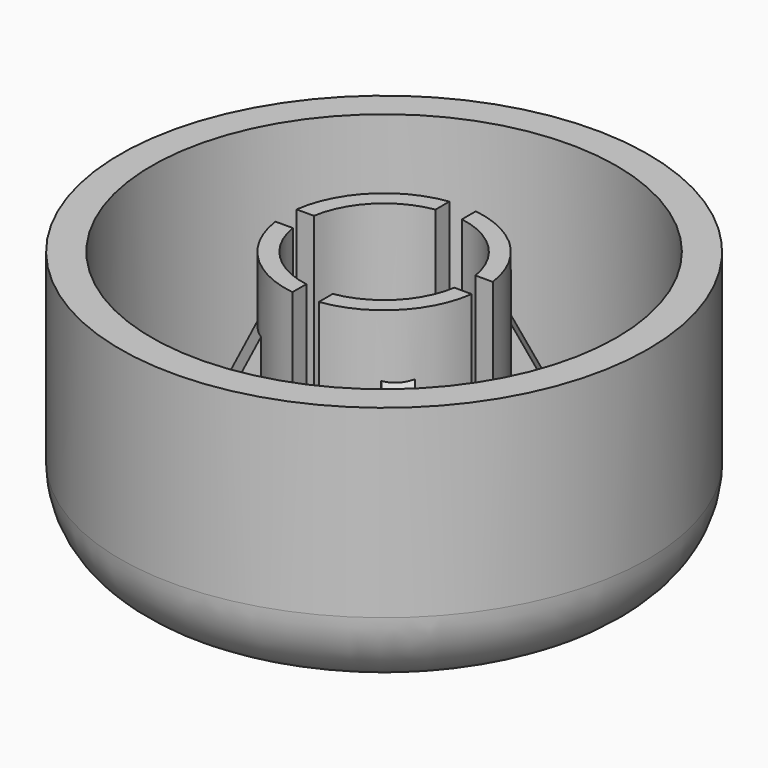
from build123d import *

# Parameters (mm, degrees)
F0_R         = 10
F0_R_2       = 3.1
F1_DEPTH     = 10
F2_R         = 8.8088832383
F2_R_2       = 3.75
F3_DEPTH     = 8
F4_W         = 1
F4_H         = 3.2863240922
F4_W_2       = 2.5055953301
F4_H_2       = 1
F5_DEPTH     = 7.5
F6_R         = 3
F8_DEPTH     = 6
F9_T4_DEPTH  = 1
F9_S5_R      = 3.75
F9_T6_DEPTH  = 5
F9_T10_DEPTH = 1
F9_S11_R     = 3.75
F9_T12_DEPTH = 5
F9_T16_DEPTH = 1
F9_S17_R     = 3.75
F9_T18_DEPTH = 5
F9_T22_DEPTH = 1
F9_S23_R     = 3.75
F9_T24_DEPTH = 5


# Not quite as in the source:
# - a fillet or chamfer that OpenCascade refuses, or shapes differently, is made with other operations: its cross-section is extruded or revolved along the edge and cut away or added
# - two fillets or chamfers of one size are made in one step


with BuildPart() as f1:
    # F0 (on Top) → F1 (new body)
    with BuildSketch(Plane.XY):
        Circle(F0_R)
        Circle(F0_R_2, mode=Mode.SUBTRACT)
    extrude(amount=F1_DEPTH)

    # F2 (on face) → F3 (cut)
    with BuildSketch(Plane.XY.offset(10)):
        Circle(F2_R)
        Circle(F2_R_2, mode=Mode.SUBTRACT)
    extrude(amount=-F3_DEPTH, mode=Mode.SUBTRACT)

    # F4 (on face) → F5 (cut)
    with BuildSketch(Plane.XY.offset(10)):
        Polygon((-2.7353764913, 0.5), (-4.8153767841, 0.5), (-4.8553765493, -0.5), (-2.7353764913, -0.5), align=None)
        Polygon((-0.5, 4.8884870484), (-0.5, 4.6887658536), (-0.5, 1.9834490959), (0.5, 1.9834490959), (0.5, 4.8884870484), align=None)
        with Locations((0, -3.2546973671)):
            Rectangle(F4_W, F4_H)
        with Locations((3.5874212626, 0)):
            Rectangle(F4_W_2, F4_H_2)
    extrude(amount=-F5_DEPTH, mode=Mode.SUBTRACT)

    # F6
    f6_edges = [f1.edges().sort_by_distance(p)[0] for p in [
        (-10, 0, 0),
    ]]
    fillet(f6_edges, radius=F6_R)

    # F7 (on face) → F8 (join)
    with BuildSketch(Plane.XY.offset(2)):
        Polygon((-4.9753358018, 4.2682290206), (-2.9815278958, 2.2744211146), (-2.2744211146, 2.9815278958), (-4.2682290206, 4.9753358018), align=None)
        Polygon((2.2744211146, 2.9815278958), (2.9815278958, 2.2744211146), (4.9753358018, 4.2682290206), (4.2682290206, 4.9753358018), align=None)
        Polygon((-2.2744211146, -2.9815278958), (-2.9815278958, -2.2744211146), (-4.9753358018, -4.2682290206), (-4.2682290206, -4.9753358018), align=None)
        Polygon((2.9815278958, -2.2744211146), (2.2744211146, -2.9815278958), (4.2682290206, -4.9753358018), (4.9753358018, -4.2682290206), align=None)
    extrude(amount=F8_DEPTH)

    # F9: chamfer of 6 x 3 on 4 edges, made by hand


with BuildPart() as f9_tool2:
    # F9_s3 → F9_t4 (new body)
    with BuildSketch(Plane(origin=(0.3535533906, 0.3535533906, 0), x_dir=(0, 0, 1), z_dir=(-0.7071067812, -0.7071067812, 0))):
        Polygon((2, 6.5361873683), (8, 3.5361873683), (8, 6.5361873683), align=None)
    extrude(amount=F9_T4_DEPTH)

    # F9_s5 → F9_t6 (cut, symmetric)
    with BuildSketch(Plane.XY.offset(5)):
        Circle(F9_S5_R)
    extrude(amount=F9_T6_DEPTH, both=True, mode=Mode.SUBTRACT)


with BuildPart() as f1_1:
    add(f1.part)

    # F9_t1: cut F9_tool2
    add(f9_tool2.part, mode=Mode.SUBTRACT)


with BuildPart() as f9_tool8:
    # F9_s9 → F9_t10 (new body)
    with BuildSketch(Plane(origin=(-0.3535533906, -0.3535533906, 0), x_dir=(0, 0, 1), z_dir=(0.7071067812, 0.7071067812, 0))):
        Polygon((2, 6.5361873683), (8, 3.5361873683), (8, 6.5361873683), align=None)
    extrude(amount=F9_T10_DEPTH)

    # F9_s11 → F9_t12 (cut, symmetric)
    with BuildSketch(Plane.XY.offset(5)):
        Circle(F9_S11_R)
    extrude(amount=F9_T12_DEPTH, both=True, mode=Mode.SUBTRACT)


with BuildPart() as f1_2:
    add(f1_1.part)

    # F9_t7: cut F9_tool8
    add(f9_tool8.part, mode=Mode.SUBTRACT)


with BuildPart() as f9_tool14:
    # F9_s15 → F9_t16 (new body)
    with BuildSketch(Plane(origin=(0.3535533906, -0.3535533906, 0), x_dir=(0, 0, 1), z_dir=(-0.7071067812, 0.7071067812, 0))):
        Polygon((2, 6.5361873683), (8, 3.5361873683), (8, 6.5361873683), align=None)
    extrude(amount=F9_T16_DEPTH)

    # F9_s17 → F9_t18 (cut, symmetric)
    with BuildSketch(Plane.XY.offset(5)):
        Circle(F9_S17_R)
    extrude(amount=F9_T18_DEPTH, both=True, mode=Mode.SUBTRACT)


with BuildPart() as f1_3:
    add(f1_2.part)

    # F9_t13: cut F9_tool14
    add(f9_tool14.part, mode=Mode.SUBTRACT)


with BuildPart() as f9_tool20:
    # F9_s21 → F9_t22 (new body)
    with BuildSketch(Plane(origin=(-0.3535533906, 0.3535533906, 0), x_dir=(0, 0, 1), z_dir=(0.7071067812, -0.7071067812, 0))):
        Polygon((2, 6.5361873683), (8, 3.5361873683), (8, 6.5361873683), align=None)
    extrude(amount=F9_T22_DEPTH)

    # F9_s23 → F9_t24 (cut, symmetric)
    with BuildSketch(Plane.XY.offset(5)):
        Circle(F9_S23_R)
    extrude(amount=F9_T24_DEPTH, both=True, mode=Mode.SUBTRACT)


with BuildPart() as f1_4:
    add(f1_3.part)

    # F9_t19: cut F9_tool20
    add(f9_tool20.part, mode=Mode.SUBTRACT)


solid = f1_4.part
